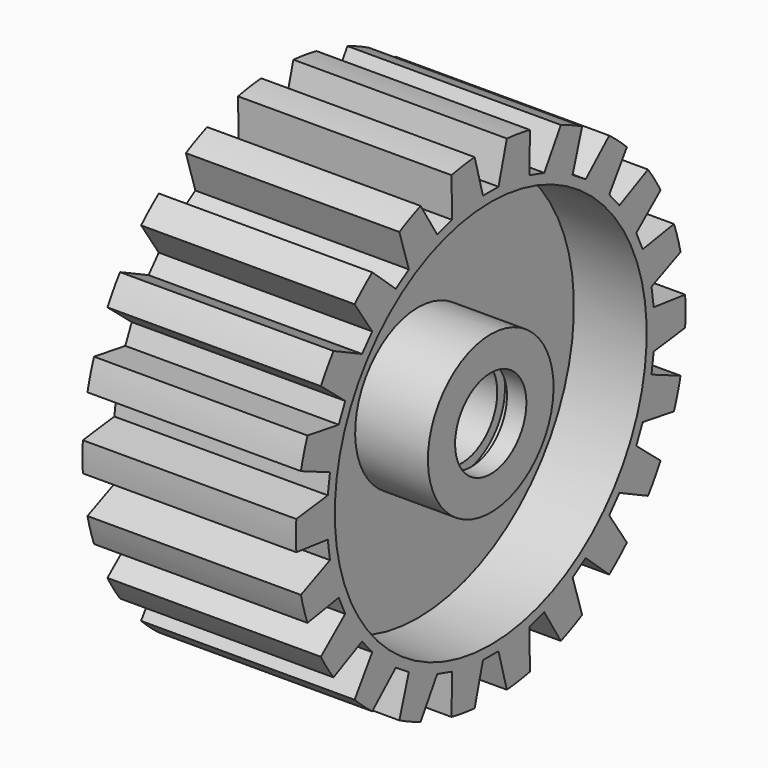
from build123d import *

# Parameters (mm, degrees)
F3_DEPTH        = 48.6
F3_COPIES_COUNT = 22


# Not quite as in the source:
# - a pattern or mirror of a feature is missing from the dataset's text; its kind, count and spacing are read off the source's solid


with BuildPart() as f1:
    # F0 (on Front) → F1 (revolve)
    with BuildSketch(Plane.XZ):
        Polygon((22, 50.1841045916), (0, 50.1841045916), (-22, 50.1841045916), (-22, 40.1841045916), (-7, 40.1841045916), (-7, 16.1841045916), (-22, 16.1841045916), (-22, 9.1841045916), (-18, 9.1841045916), (-18, 11.1841045916), (-16, 11.1841045916), (-16, 9.1841045916), (-1.5, 9.1841045916), (-1.5, 7.1841045916), (0, 7.1841045916), (1.5, 7.1841045916), (1.5, 9.1841045916), (16, 9.1841045916), (16, 11.1841045916), (18, 11.1841045916), (18, 9.1841045916), (22, 9.1841045916), (22, 16.1841045916), (7, 16.1841045916), (7, 40.1841045916), (22, 40.1841045916), align=None)
    revolve(axis=Axis((-7.0416135713, 0, 0), (-1, 0, 0)))

    # F2 (on Right) → F3 (cut, symmetric)
    with BuildSketch(Plane.YZ):
        Polygon((-2, 42.1328544021), (0, 42.1328544021), (2, 42.1328544021), (5, 53.1328544021), (0, 53.1328544021), (-5, 53.1328544021), align=None)
    f3 = extrude(amount=F3_DEPTH, both=True, mode=Mode.SUBTRACT)

    # F3_copies: F3 ×22 about axis
    f3_copies_axis = Axis((0, 0, 0), (1, 0, 0))
    for i in range(1, F3_COPIES_COUNT):
        add(f3.rotate(f3_copies_axis, i * 360 / F3_COPIES_COUNT), mode=Mode.SUBTRACT)


solid = f1.part
